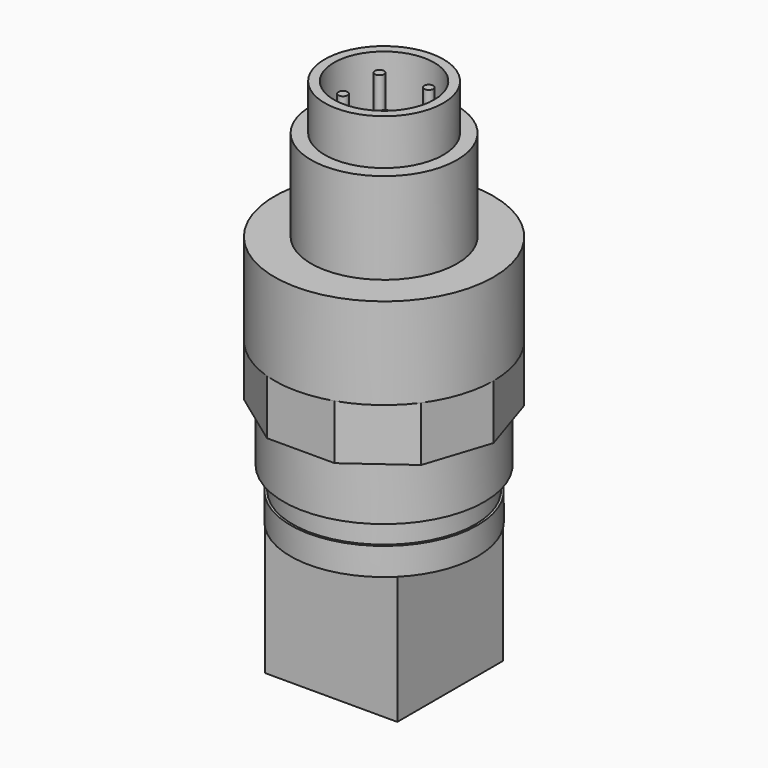
from build123d import *

# Parameters (mm, degrees)
F0_R      = 3.25
F1_DEPTH  = 2.5
F2_R      = 4
F2_R_2    = 3.25
F3_DEPTH  = 5
F4_R      = 6
F4_R_2    = 4
F5_DEPTH  = 5
F7_DEPTH  = 3
F8_R      = 5.5
F9_DEPTH  = 3
F10_R     = 5
F11_DEPTH = 1.25
F12_R     = 5.125
F12_R_2   = 5
F13_DEPTH = 1.5
F14_W     = 7.2478445072
F14_H     = 7.2478445072
F15_DEPTH = 7
F16_R     = 2.75
F17_DEPTH = 5
F18_R     = 0.25
F19_DEPTH = 4.5


with BuildPart() as f1:
    # F0 (on Top) → F1 (new body)
    with BuildSketch(Plane.XY):
        Circle(F0_R)
    extrude(amount=-F1_DEPTH)

    # F2 (on face) → F3 (join)
    with BuildSketch(Plane(origin=(0, 0, -2.5), x_dir=(1, 0, 0), z_dir=(0, 0, -1))):
        Circle(F2_R)
        Circle(F2_R_2, mode=Mode.SUBTRACT)
        Circle(F2_R_2)
    extrude(amount=F3_DEPTH)

    # F4 (on face) → F5 (join)
    with BuildSketch(Plane(origin=(0, 0, -7.5), x_dir=(1, 0, 0), z_dir=(0, 0, -1))):
        Circle(F4_R)
        Circle(F4_R_2, mode=Mode.SUBTRACT)
        Circle(F4_R_2)
    extrude(amount=F5_DEPTH)

    # F6 (on face) → F7 (join)
    with BuildSketch(Plane(origin=(0, 0, -12.5), x_dir=(1, 0, 0), z_dir=(0, 0, -1))):
        Polygon((4.8541019662, -3.5267115138), (6, 0), (4.8541019662, 3.5267115138), (1.8541019662, 5.7063390978), (-1.8541019662, 5.7063390978), (-4.8541019662, 3.5267115138), (-6, 0), (-4.8541019662, -3.5267115138), (-1.8541019662, -5.7063390978), (1.8541019662, -5.7063390978), align=None)
    extrude(amount=F7_DEPTH)

    # F8 (on face) → F9 (join)
    with BuildSketch(Plane(origin=(0, 0, -15.5), x_dir=(1, 0, 0), z_dir=(0, 0, -1))):
        Circle(F8_R)
    extrude(amount=F9_DEPTH)

    # F10 (on face) → F11 (join)
    with BuildSketch(Plane(origin=(0, 0, -18.5), x_dir=(1, 0, 0), z_dir=(0, 0, -1))):
        Circle(F10_R)
    extrude(amount=F11_DEPTH)

    # F12 (on face) → F13 (join)
    with BuildSketch(Plane(origin=(0, 0, -19.75), x_dir=(1, 0, 0), z_dir=(0, 0, -1))):
        Circle(F12_R)
        Circle(F12_R_2, mode=Mode.SUBTRACT)
        Circle(F12_R_2)
    extrude(amount=F13_DEPTH)

    # F14 (on face) → F15 (join)
    with BuildSketch(Plane(origin=(0, 0, -21.25), x_dir=(1, 0, 0), z_dir=(0, 0, -1))):
        Rectangle(F14_W, F14_H)
    extrude(amount=F15_DEPTH)

    # F16 (on face) → F17 (cut)
    with BuildSketch(Plane.XY):
        Circle(F16_R)
    extrude(amount=-F17_DEPTH, mode=Mode.SUBTRACT)

    # F18 (on face) → F19 (join)
    with BuildSketch(Plane.XY.offset(-5)):
        with Locations((-1.25, -1.25)):
            Circle(F18_R)
        with Locations((1.25, -1.5)):
            Circle(F18_R)
        with Locations((1.25, 1.5)):
            Circle(F18_R)
        with Locations((-1.25, 1.25)):
            Circle(F18_R)
    extrude(amount=F19_DEPTH)


solid = f1.part
